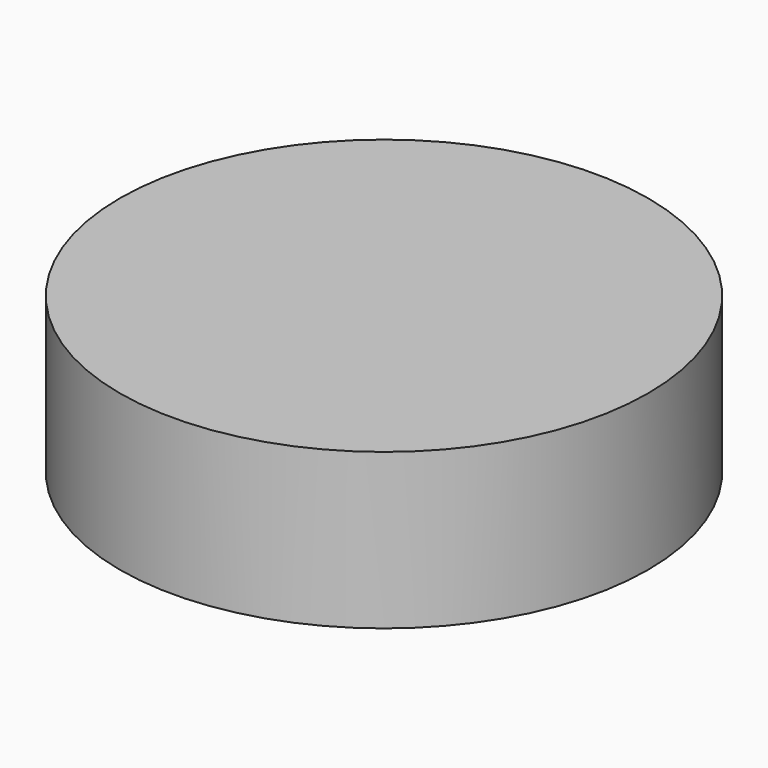
from build123d import *

# Parameters (mm, degrees)
F0_R     = 8.5
F1_DEPTH = 5


# Not quite as in the source:
# - the program builds the solid bodies; features that only make, move or delete a surface that nothing else refers to are left out


with BuildPart() as f1:
    # F0 (on Top) → F1 (new body)
    with BuildSketch(Plane.XY):
        Circle(F0_R)
    extrude(amount=F1_DEPTH)


solid = f1.part
